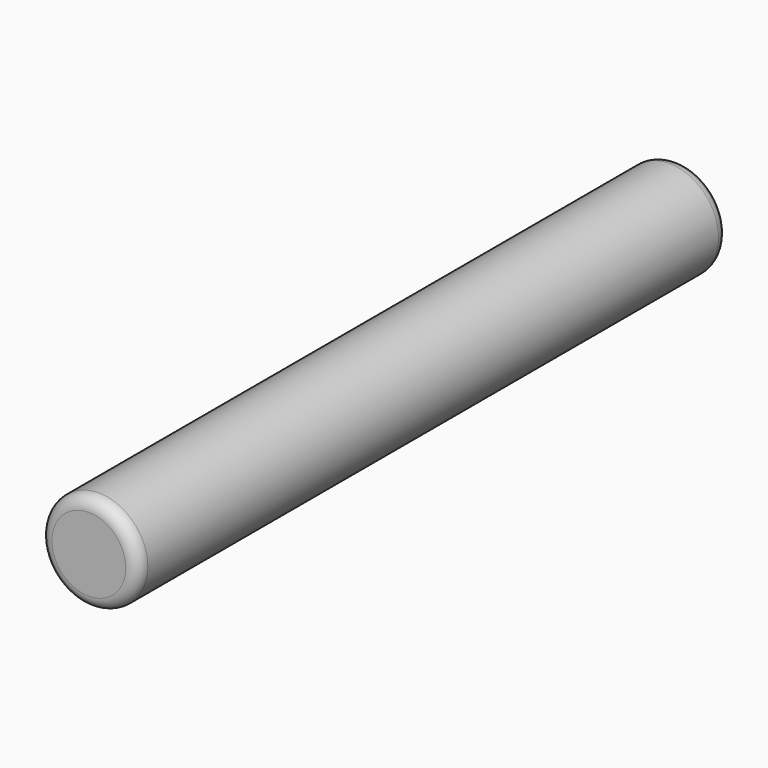
from build123d import *

# Parameters (mm, degrees)
F2_R = 0.5


with BuildPart() as f1:
    # F0 (on Right) → F1 (revolve)
    with BuildSketch(Plane.YZ):
        Polygon((-11.0091740638, 11.247707203), (-15.0091740638, 11.247707203), (-22.9062791914, 11.247707203), (-23.5091740638, 11.247707203), (-28.5091740638, 11.247707203), (-28.8583226502, 11.247707203), (-29.1120689362, 11.247707203), (-37.0091740638, 11.247707203), (-41.0091740638, 11.247707203), (-41.0091740638, 9.247707203), (-26.0091740638, 9.247707203), (-11.0091740638, 9.247707203), align=None)
    revolve(axis=Axis((0, -26.3120413944, 9.247707203), (0, 1, 0)))

    # F2
    f2_edges = [f1.edges().sort_by_distance(p)[0] for p in [
        (0, -41.009174, 7.247707),
        (0, -11.009174, 7.247707),
    ]]
    fillet(f2_edges, radius=F2_R)


solid = f1.part
